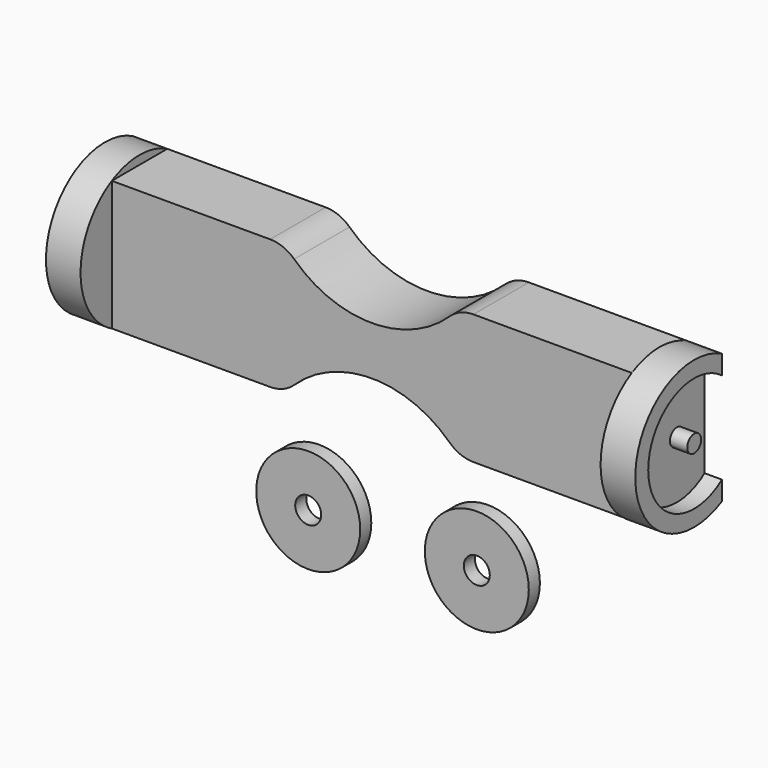
from build123d import *

# Parameters (mm, degrees)
F1_DEPTH  = 10.16
F2_W      = 10.16
F2_H      = 19.05
F3_DEPTH  = 5.08
F5_DEPTH  = 2.54
F6_W      = 10.16
F6_H      = 19.05
F7_DEPTH  = 5.08
F9_DEPTH  = 2.54
F10_R     = 1.27
F11_DEPTH = 2.54
F12_R     = 1.27
F13_DEPTH = 2.54
F14_R     = 7.62
F14_R_2   = 1.905
F15_DEPTH = 2.032
F16_R     = 5.08


with BuildPart() as f1:
    # F0 (on Front) → F1 (new body)
    with BuildSketch(Plane.XZ):
        with BuildLine():
            Line((-21.5824204445, 9.525), (-46.9824204445, 9.525))
            Line((-46.9824204445, 9.525), (-46.9824204445, -9.525))
            Line((-46.9824204445, -9.525), (-21.5824204445, -9.525))
            ThreePointArc((-21.5824204445, -9.525), (-8.8824204445, -3.5644123059), (3.8175795555, -9.525))
            Line((3.8175795555, -9.525), (29.2175795555, -9.525))
            Line((29.2175795555, -9.525), (29.2175795555, 9.525))
            Line((29.2175795555, 9.525), (3.8175795555, 9.525))
            ThreePointArc((3.8175795555, 9.525), (-8.8824204445, 3.5644123059), (-21.5824204445, 9.525))
        make_face()
    extrude(amount=F1_DEPTH)

    # F2 (on face) → F3 (join)
    with BuildSketch(Plane.YZ.offset(29.2175795555)):
        with BuildLine():
            Line((-10.16, 9.525), (0, 9.525))
            ThreePointArc((0, 9.525), (-5.08, 10.795), (-10.16, 9.525))
        make_face()
        with Locations((-5.08, 0)):
            Rectangle(F2_W, F2_H)
        with BuildLine():
            ThreePointArc((-10.16, -9.525), (-5.08, -10.795), (0, -9.525))
            Line((0, -9.525), (-10.16, -9.525))
        make_face()
        with BuildLine():
            Line((-10.16, -9.525), (-10.16, 9.525))
            ThreePointArc((-10.16, 9.525), (-15.875, 0), (-10.16, -9.525))
        make_face()
    extrude(amount=F3_DEPTH)

    # F4 (on face) → F5 (cut)
    with BuildSketch(Plane.YZ.offset(34.2975795555)):
        with BuildLine():
            Line((0, -6.7160268108), (0, 6.7160268108))
            ThreePointArc((0, 6.7160268108), (-13.5008916466, 0), (0, -6.7160268108))
        make_face()
    extrude(amount=-F5_DEPTH, mode=Mode.SUBTRACT)

    # F6 (on face) → F7 (join)
    with BuildSketch(Plane(origin=(-46.9824204445, 0, 0), x_dir=(0, -1, 0), z_dir=(-1, 0, 0))):
        with BuildLine():
            Line((10.16, -9.525), (0, -9.525))
            ThreePointArc((0, -9.525), (15.8755169753, 0), (0, 9.525))
            Line((0, 9.525), (10.16, 9.525))
            Line((10.16, 9.525), (10.16, -9.525))
        make_face()
        with Locations((5.08, 0)):
            Rectangle(F6_W, F6_H)
    extrude(amount=F7_DEPTH)

    # F8 (on face) → F9 (cut)
    with BuildSketch(Plane(origin=(-52.0624204445, 0, 0), x_dir=(0, -1, 0), z_dir=(-1, 0, 0))):
        with BuildLine():
            ThreePointArc((0, -6.6626255848), (8.7975033543, -7.5088836617), (13.4589284751, 0))
            ThreePointArc((13.4589284751, 0), (8.7975033543, 7.5088836617), (0, 6.6626255848))
            Line((0, 6.6626255848), (0, -6.6626255848))
        make_face()
    extrude(amount=-F9_DEPTH, mode=Mode.SUBTRACT)

    # F10 (on face) → F11 (join)
    with BuildSketch(Plane.YZ.offset(31.7575795555)):
        with Locations((-5.08, 0)):
            Circle(F10_R)
    extrude(amount=F11_DEPTH)

    # F12 (on face) → F13 (join)
    with BuildSketch(Plane(origin=(-49.5224204445, 0, 0), x_dir=(0, -1, 0), z_dir=(-1, 0, 0))):
        with Locations((5.0803515401, 0)):
            Circle(F12_R)
    extrude(amount=F13_DEPTH)

    # F16
    f16_edges = [f1.edges().sort_by_distance(p)[0] for p in [
        (-21.58242, -5.08, 9.525),
        (3.81758, -5.08, 9.525),
        (3.81758, -5.08, -9.525),
        (-21.58242, -5.08, -9.525),
    ]]
    fillet(f16_edges, radius=F16_R)


with BuildPart() as f15:
    # F14 (on Front) → F15 (new body)
    with BuildSketch(Plane.XZ):
        with Locations((0, -28.7541169673)):
            Circle(F14_R)
        with Locations((0, -28.7541169673)):
            Circle(F14_R_2, mode=Mode.SUBTRACT)
    extrude(amount=F15_DEPTH)


with BuildPart() as f15b:
    # F14 (on Front) → F15, piece 2 (new body)
    with BuildSketch(Plane.XZ):
        with Locations((-24.7039161623, -29.0205683559)):
            Circle(F14_R)
        with Locations((-24.7039161623, -29.0205683559)):
            Circle(F14_R_2, mode=Mode.SUBTRACT)
    extrude(amount=F15_DEPTH)


solid = Compound([f1.part, f15.part, f15b.part])
